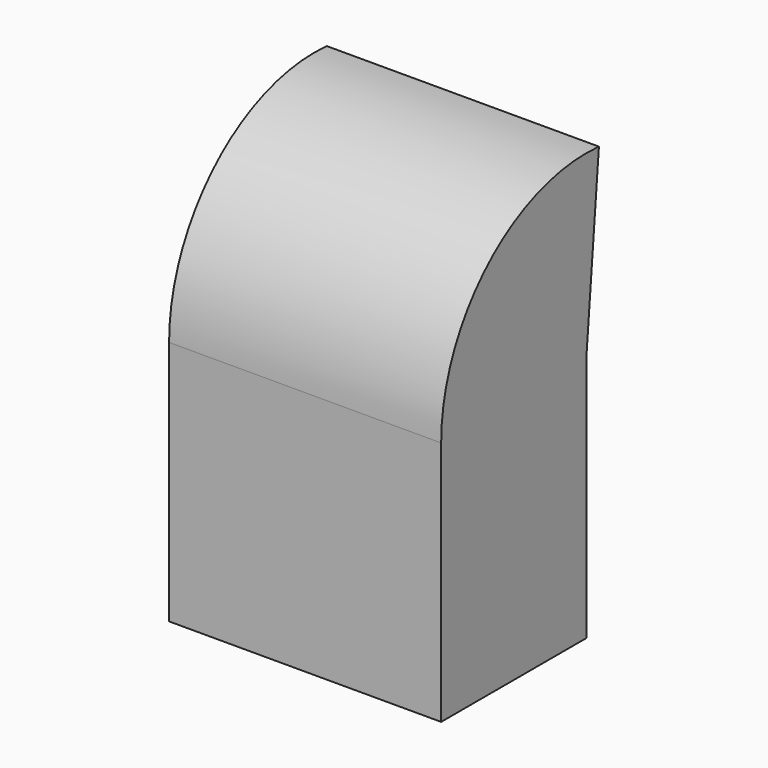
from build123d import *

# Parameters (mm, degrees)
F2_W     = 914.4
F2_H     = 609.6
F3_DEPTH = 825.5
F4_W     = 914.4
F4_H     = 609.6
F5_ANGLE = 95


# Not quite as in the source:
# - a variable given as a bare number and used for a length is read in inches; the dataset says mm whatever the document's units were


with BuildPart() as f3:
    # F2 (on Top) → F3 (new body)
    with BuildSketch(Plane.XY):
        Rectangle(F2_W, F2_H)
    extrude(amount=F3_DEPTH)

    # F4 (on face) → F5 (revolve)
    with BuildSketch(Plane.XY.offset(825.5)):
        Rectangle(F4_W, F4_H)
    revolve(axis=Axis((0, 304.8, 825.5), (-1, 0, 0)), revolution_arc=F5_ANGLE)


solid = f3.part
